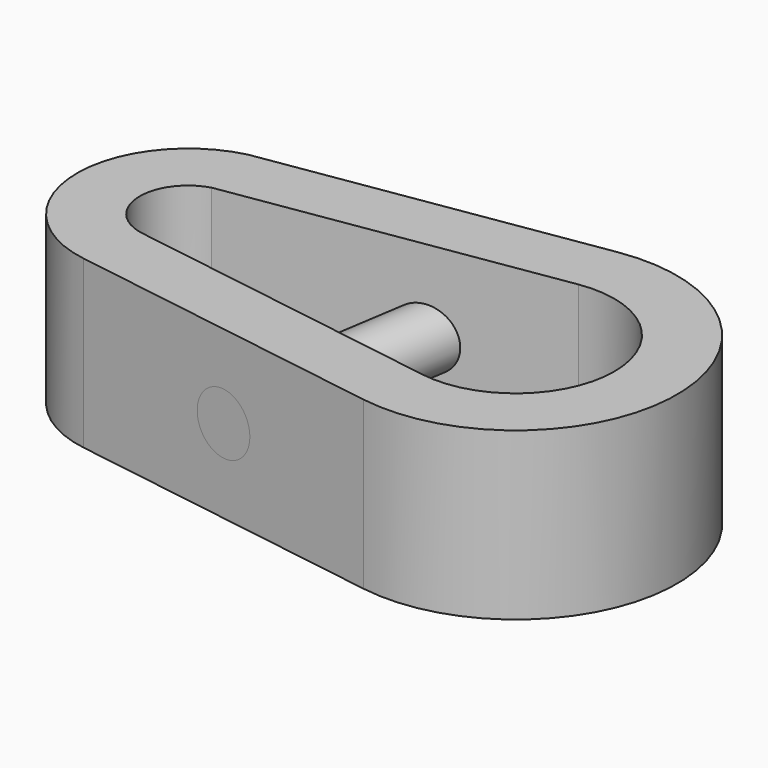
from build123d import *

# Parameters (mm, degrees)
F1_DEPTH = 53.2
F2_R     = 9.7217056973
F3_DEPTH = 106.8
F4_DEPTH = 33.4


# Not quite as in the source:
# - ends of sketch curves that miss each other by under 0.0002 mm in the source are joined


with BuildPart() as f1:
    # F0 (on Top) → F1 (new body)
    with BuildSketch(Plane.XY):
        with BuildLine():
            Line((-7.9474923426, 50.9009919427), (-113.0345375872, 34.4224307572))
            ThreePointArc((-113.0345375872, 34.4224307572), (-140.0579018259, -1.5509775623), (-109.9911685167, -35.0224560031))
            Line((-109.9911685167, -35.0224560031), (-7.9210999462, -50.905094516))
            ThreePointArc((-7.9210999462, -50.905094516), (51.5176891338, 0.0133546718), (-7.9474923426, 50.9009919427))
        make_face()
        with BuildLine():
            ThreePointArc((-4.8825833147, 31.1371999002), (31.5176854276, 0.01851299), (-4.8460009605, -31.1429143167))
            Line((-4.8460009605, -31.1429143167), (-106.957762942, -15.2537880902))
            ThreePointArc((-106.957762942, -15.2537880902), (-120.0581940893, -1.0187143376), (-108.9482164871, 14.8188049967))
            Line((-108.9482164871, 14.8188049967), (-4.8825833147, 31.1371999002))
        make_face(mode=Mode.SUBTRACT)
    extrude(amount=-F1_DEPTH)

    # F2 (on face) → F3 (join)
    with BuildSketch(Plane(origin=(-7.9210999462, -50.905094516, 0), x_dir=(0.98810901, -0.1537549493, 0), z_dir=(-0.1537549493, -0.98810901, 0))):
        with Locations((-51.6491943406, -26.6)):
            Circle(F2_R)
    extrude(amount=-F3_DEPTH)

    # F4 (add): a face of the model
    f4_faces = [f1.faces().sort_by_distance(p)[0] for p in [
        (-42.5351056478, 62.5662670045, -26.6),
    ]]
    extrude(f4_faces, amount=-F4_DEPTH)


solid = f1.part
